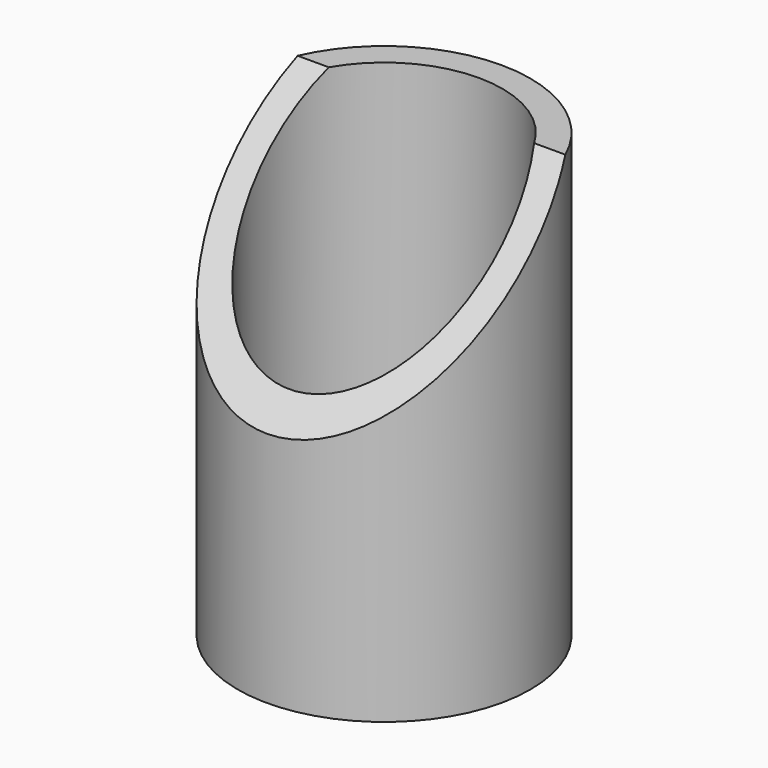
from build123d import *

# Parameters (mm, degrees)
F0_R     = 21
F0_R_2   = 17
F1_DEPTH = 63.5
F3_DEPTH = 21


# Not quite as in the source:
# - a feature names something its author has since deleted; it is built from what else it names


with BuildPart() as f1:
    # F0 (on Top) → F1 (new body)
    with BuildSketch(Plane.XY):
        Circle(F0_R)
        Circle(F0_R_2, mode=Mode.SUBTRACT)
    extrude(amount=F1_DEPTH)

    # F2 (on Right) → F3 (cut, symmetric)
    with BuildSketch(Plane.YZ):
        Polygon((-21, 34), (8.5, 63.5), (21, 63.5), (21, 73.5), (-21, 73.5), align=None)
        Polygon((21, -63.5), (8.5, -63.5), (-21, -34), (-21, -73.5), (21, -73.5), align=None)
    extrude(amount=F3_DEPTH, both=True, mode=Mode.SUBTRACT)


solid = f1.part
